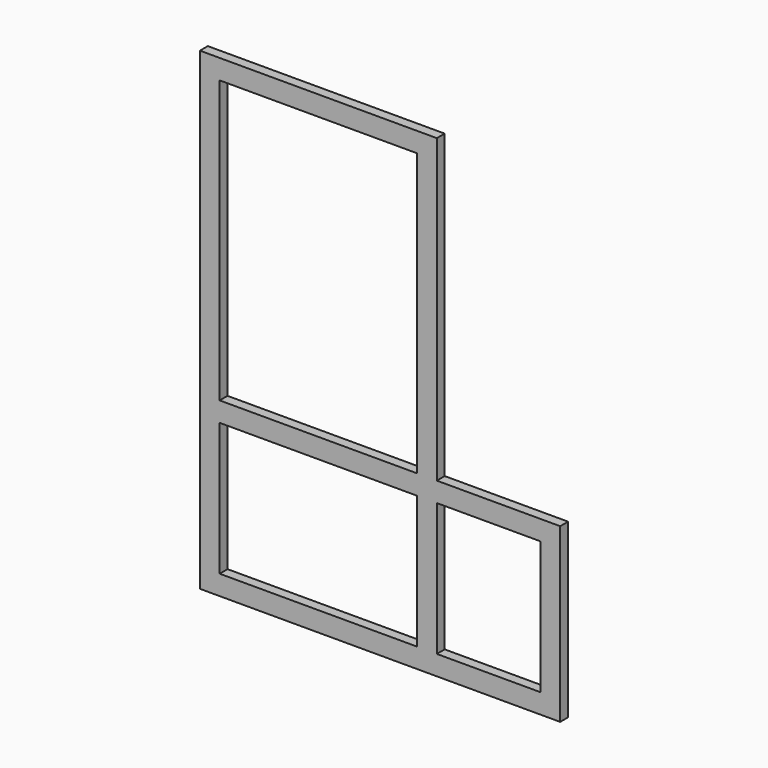
from build123d import *

# Parameters (mm, degrees)
F0_W     = 800
F0_H     = 80
F1_DEPTH = 40
F0_W_2   = 420
F0_W_3   = 80
F0_H_2   = 538.2458400726
F2_DEPTH = 40
F3_DEPTH = 40


# Not quite as in the source:
# - a feature names something its author has since deleted; it is built from what else it names


with BuildPart() as f1:
    # F0 (on Front) → F1 (new body)
    with BuildSketch(Plane.XZ):
        with Locations((400, 1800)):
            Rectangle(F0_W, F0_H)
        Polygon((-80, 1840), (-80, -80), (0, -80), (0, 0), (0, 538.2458400726), (0, 618.2458400726), (0, 1760), (0, 1840), align=None)
        with Locations((400, -40)):
            Rectangle(F0_W, F0_H)
        Polygon((800, 0), (800, -80), (880, -80), (880, 0), (880, 538.2458400726), (880, 618.2458400726), (880, 1840), (800, 1840), (800, 1760), (800, 618.2458400726), (800, 538.2458400726), align=None)
    extrude(amount=F1_DEPTH)

    # F0 (on Front) → F2 (join)
    with BuildSketch(Plane.XZ):
        Polygon((-80, 1840), (-80, -80), (0, -80), (0, 0), (0, 538.2458400726), (0, 618.2458400726), (0, 1760), (0, 1840), align=None)
        with Locations((400, -40)):
            Rectangle(F0_W, F0_H)
        with Locations((400, 1800)):
            Rectangle(F0_W, F0_H)
        Polygon((800, 0), (800, -80), (880, -80), (880, 0), (880, 538.2458400726), (880, 618.2458400726), (880, 1840), (800, 1840), (800, 1760), (800, 618.2458400726), (800, 538.2458400726), align=None)
        Polygon((880, 0), (880, -80), (1380, -80), (1380, 0), (1300, 0), align=None)
        with Locations((1090, 578.2458400726)):
            Rectangle(F0_W_2, F0_H)
        with Locations((1340, 269.1229200363)):
            Rectangle(F0_W_3, F0_H_2)
        with Locations((1340, 578.2458400726)):
            Rectangle(F0_W_3, F0_H)
    extrude(amount=F2_DEPTH)

    # F0 (on Front) → F3 (join)
    with BuildSketch(Plane.XZ):
        with Locations((400, 578.2458400726)):
            Rectangle(F0_W, F0_H)
    extrude(amount=F3_DEPTH)


solid = f1.part
